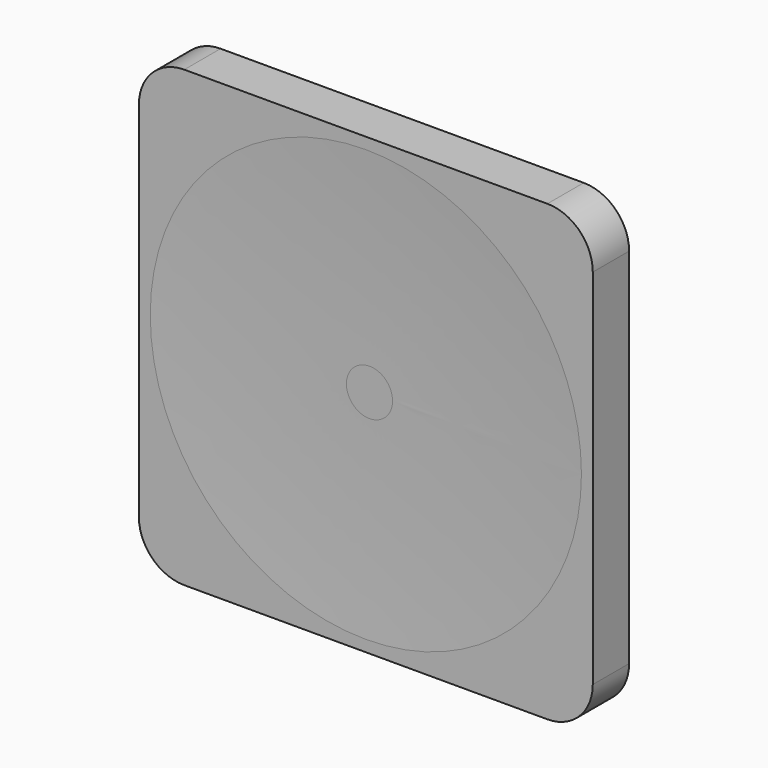
from build123d import *

# Parameters (mm, degrees)
F0_W     = 50.8
F0_H     = 50.8
F1_DEPTH = 5.08
F2_W     = 9.525
F2_H     = 9.525
F2_W_2   = 3.048
F2_H_2   = 3.048
F3_DEPTH = 12.7
F4_R     = 5.08
F5_R     = 5.08
F6_R     = 24.13
F7_DEPTH = 0.508


# Not quite as in the source:
# - a fillet or chamfer that OpenCascade refuses, or shapes differently, is made with other operations: its cross-section is extruded or revolved along the edge and cut away or added


with BuildPart() as f1:
    # F0 (on Front) → F1 (new body)
    with BuildSketch(Plane.XZ):
        Rectangle(F0_W, F0_H)
    extrude(amount=F1_DEPTH)

    # F2 (on face) → F3 (join)
    with BuildSketch(Plane(origin=(0, 0, 0), x_dir=(-1, 0, 0), z_dir=(0, 1, 0))):
        Rectangle(F2_W, F2_H)
        Rectangle(F2_W_2, F2_H_2, mode=Mode.SUBTRACT)
    extrude(amount=F3_DEPTH)

    # F4
    f4_edges = [f1.edges().sort_by_distance(p)[0] for p in [
        (0, 0, -4.7625),
        (-4.7625, 0, 0),
        (4.7625, 0, 0),
        (0, 0, 4.7625),
    ]]
    fillet(f4_edges, radius=F4_R)

    # F5
    f5_edges = [f1.edges().sort_by_distance(p)[0] for p in [
        (-25.4, -2.54, 25.4),
        (-25.4, -2.54, -25.4),
        (25.4, -2.54, 25.4),
        (25.4, -2.54, -25.4),
    ]]
    fillet(f5_edges, radius=F5_R)

    # F6 (on face) → F7 (cut)
    with BuildSketch(Plane.XZ.offset(5.08)):
        Circle(F6_R)
    extrude(amount=-F7_DEPTH, mode=Mode.SUBTRACT)

    # F8: fillet of radius 457.2 on 1 edges, made by hand

    # F8_s1 → F8_t2 (revolve)
    with BuildSketch(Plane.XY):
        with BuildLine():
            ThreePointArc((24.13, -5.08), (13.3596803239, -4.6990176438), (2.5833729786, -4.572))
            Line((2.5833729786, -4.572), (24.13, -4.572))
            Line((24.13, -4.572), (24.13, -5.08))
        make_face()
    revolve(axis=Axis((0, -4.572, 0), (0, -1, 0)))


solid = f1.part
